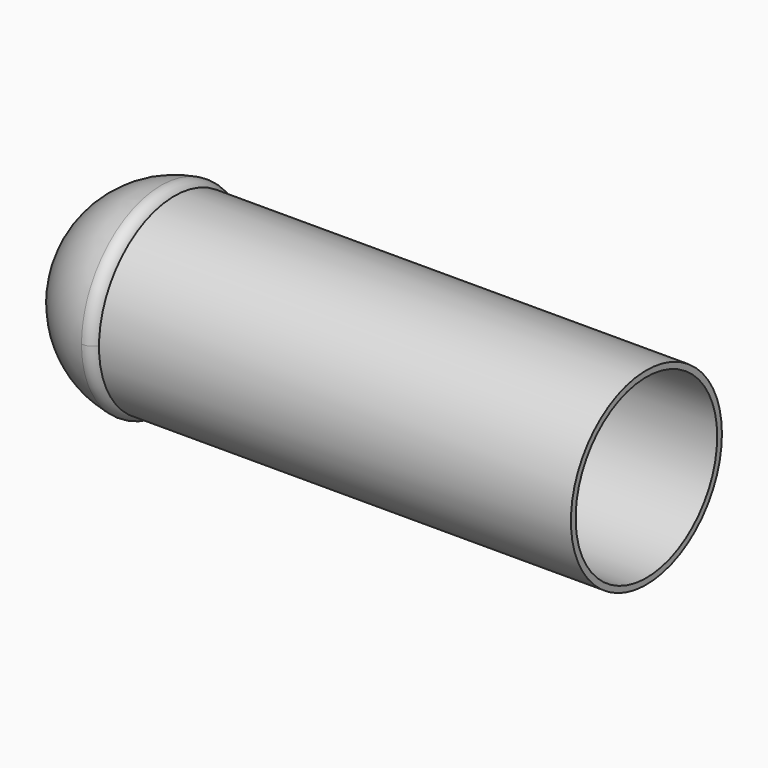
from build123d import *
from build123d import SkipClean  # not in build123d's __all__

# Parameters (mm, degrees)
F1_ANGLE    = 180
F2_R        = 15
F3_DEPTH    = 30
F4_R        = 16
F4_R_2      = 15
F5_DEPTH    = 80
F6_T2_ANGLE = 180
F6_T4_ANGLE = 180


# Not quite as in the source:
# - a fillet or chamfer that OpenCascade refuses, or shapes differently, is made with other operations: its cross-section is extruded or revolved along the edge and cut away or added


with BuildPart() as f1:
    # F0 (on Right) → F1 (revolve)
    with BuildSketch(Plane.YZ):
        with BuildLine():
            Line((30.0467135459, -7.373497352), (-3.9532864541, -7.373497352))
            ThreePointArc((-3.9532864541, -7.373497352), (13.0467135459, -24.373497352), (30.0467135459, -7.373497352))
        make_face()
    revolve(axis=Axis((0, 13.0467135459, -7.373497352), (0, 1, 0)), revolution_arc=F1_ANGLE)

    # F2 (on face) → F3 (join)
    with BuildSketch(Plane.YZ):
        with Locations((13.0467135459, -7.373497352)):
            Circle(F2_R)
    extrude(amount=F3_DEPTH)

    # F6: fillet of radius 2 on 1 edges, made by hand

    # F6_s1 → F6_t2 (revolve, cut)
    with BuildSketch(Plane.XY.offset(-7.373497352)):
        with BuildLine():
            ThreePointArc((-2.2616240205, -3.802175343), (-0.7297029178, -3.3683812365), (0, -1.9532864541))
            Line((0, -1.9532864541), (0.0399110121, -1.9559531207))
            ThreePointArc((0.0399110121, -1.9559531207), (0.04, -2.9532864541), (0.04, -3.9532864541))
            Line((0.04, -3.9532864541), (0, -3.9932864541))
            ThreePointArc((0, -3.9932864541), (-1.136, -3.9553776196), (-2.2669454887, -3.8418197874))
            Line((-2.2669454887, -3.8418197874), (-2.2616240205, -3.802175343))
        make_face()
    revolve(axis=Axis((0, 13.0467135459, -7.373497352), (1, 0, 0)), revolution_arc=F6_T2_ANGLE, mode=Mode.SUBTRACT)

    # F6_s3 → F6_t4 (revolve, cut)
    with BuildSketch(Plane.XY.offset(-7.373497352)):
        with BuildLine():
            ThreePointArc((-2.2616240205, -3.802175343), (-0.7297029178, -3.3683812365), (0, -1.9532864541))
            Line((0, -1.9532864541), (0.0399110121, -1.9559531207))
            ThreePointArc((0.0399110121, -1.9559531207), (0.04, -2.9532864541), (0.04, -3.9532864541))
            Line((0.04, -3.9532864541), (0, -3.9932864541))
            ThreePointArc((0, -3.9932864541), (-1.136, -3.9553776196), (-2.2669454887, -3.8418197874))
            Line((-2.2669454887, -3.8418197874), (-2.2616240205, -3.802175343))
        make_face()
    with SkipClean():  # cleaning this boolean's faces spoils the solid; the shape is the same uncleaned
        revolve(axis=Axis((0, 13.0467135459, -7.373497352), (-1, 0, 0)), revolution_arc=F6_T4_ANGLE, mode=Mode.SUBTRACT)


with BuildPart() as f5:
    # F4 (on face) → F5 (new body)
    with BuildSketch(Plane.YZ):
        with Locations((13.0467135459, -7.373497352)):
            Circle(F4_R)
        with Locations((13.0467135459, -7.373497352)):
            Circle(F4_R_2, mode=Mode.SUBTRACT)
    extrude(amount=F5_DEPTH)


solid = Compound([f1.part, f5.part])
